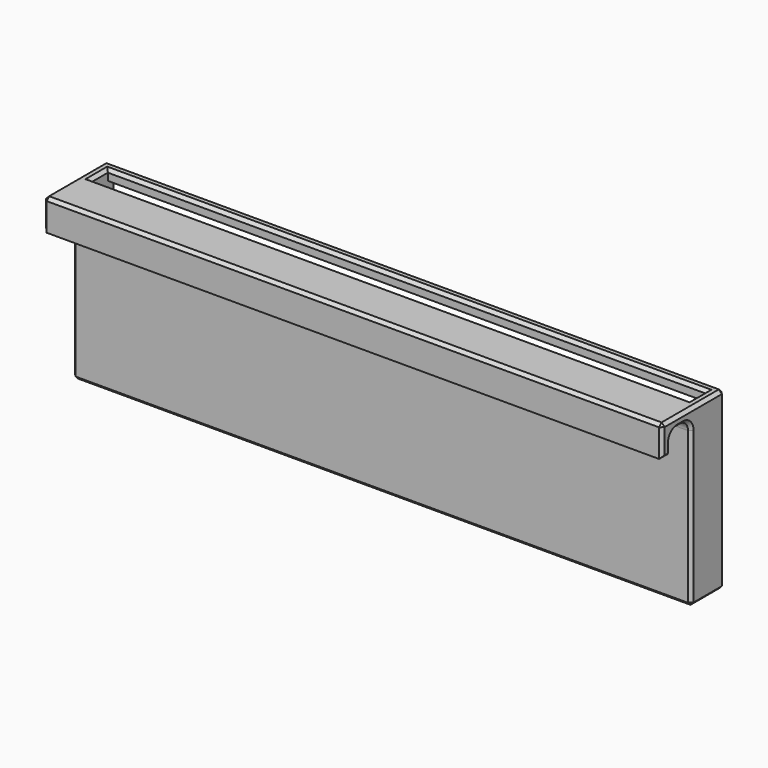
from build123d import *

# Parameters (mm, degrees)
F0_W     = 10.2
F0_H     = 75
F1_DEPTH = 300
F2_W     = 290
F2_H     = 70
F3_DEPTH = 5
F4_W     = 290
F4_H     = 10.2
F5_DEPTH = 80
F6_SIZE  = 1.5


# Not quite as in the source:
# - a feature names something its author has since deleted; it is built from what else it names


with BuildPart() as f1:
    # F0 (on Right) → F1 (new body)
    with BuildSketch(Plane.YZ):
        Polygon((-10.1, -42.5), (10.1, -42.5), (10.1, 42.5), (-27.6, 42.5), (-27.6, 27.5), (-22.6, 27.5), (-22.6, 33.5), (-22.6, 37.5), (-18.6, 37.5), (-15.1, 37.5), (-10.1, 37.5), (-10.1, 32.5), align=None)
        Rectangle(F0_W, F0_H, mode=Mode.SUBTRACT)
        with BuildLine():
            ThreePointArc((-22.6, 33.5), (-21.4284271247, 36.3284271247), (-18.6, 37.5))
            Line((-18.6, 37.5), (-22.6, 37.5))
            Line((-22.6, 37.5), (-22.6, 33.5))
        make_face()
        with BuildLine():
            ThreePointArc((-15.1, 37.5), (-11.5644660941, 36.0355339059), (-10.1, 32.5))
            Line((-10.1, 32.5), (-10.1, 37.5))
            Line((-10.1, 37.5), (-15.1, 37.5))
        make_face()
        Rectangle(F0_W, F0_H)
    extrude(amount=F1_DEPTH)

    # F2 (on face) → F3 (cut)
    with BuildSketch(Plane(origin=(0, 10.1, 0), x_dir=(-1, 0, 0), z_dir=(0, 1, 0))):
        with Locations((-150, 2.5)):
            Rectangle(F2_W, F2_H)
    extrude(amount=-F3_DEPTH, mode=Mode.SUBTRACT)

    # F4 (on face) → F5 (cut)
    with BuildSketch(Plane.XY.offset(42.5)):
        with Locations((150, 0)):
            Rectangle(F4_W, F4_H)
    extrude(amount=-F5_DEPTH, mode=Mode.SUBTRACT)

    # F6
    f6_edges = [f1.edges().sort_by_distance(p)[0] for p in [
        (300, 0, -42.5),
        (300, 10.1, 0),
        (300, -8.75, 42.5),
        (300, -27.6, 35),
        (300, -25.1, 27.5),
        (300, -22.6, 30.5),
        (300, -21.428427, 36.328427),
        (300, -16.85, 37.5),
        (300, -11.564466, 36.035534),
        (300, -10.1, -5),
        (150, 10.1, -42.5),
        (0, 10.1, 0),
        (150, 10.1, 42.5),
        (5, 10.1, 2.5),
        (150, 10.1, -32.5),
        (295, 10.1, 2.5),
        (150, 10.1, 37.5),
        (0, -8.75, 42.5),
        (150, -27.6, 42.5),
        (150, -5.1, 42.5),
        (5, 0, 42.5),
        (150, 5.1, 42.5),
        (295, 0, 42.5),
        (150, -10.1, -42.5),
        (0, 0, -42.5),
        (0, -27.6, 35),
        (0, -25.1, 27.5),
        (0, -22.6, 30.5),
        (0, -21.428427, 36.328427),
        (0, -16.85, 37.5),
        (0, -11.564466, 36.035534),
        (0, -10.1, -5),
    ]]
    chamfer(f6_edges, length=F6_SIZE)


solid = f1.part
